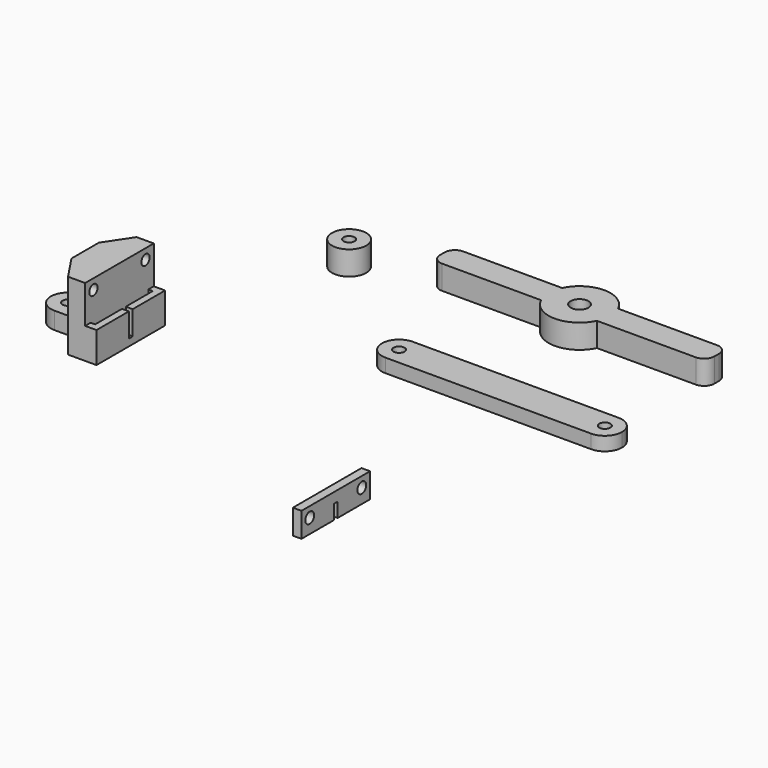
from build123d import *

# Parameters (mm, degrees)
F0_W      = 70
F0_H      = 10
F0_R      = 1.6
F1_DEPTH  = 4
F2_R      = 4.99999
F3_R      = 5
F3_R_2    = 1.6
F4_DEPTH  = 7
F7_DEPTH  = 20
F6_W      = 10
F6_H      = 10
F8_DEPTH  = 5
F10_D     = 3.2
F10_DEPTH = 5
F10_TIP   = 0.9613769904
F11_R     = 4.99999
F13_DEPTH = 1.3
F14_W     = 9.8
F14_H     = 7
F15_DEPTH = 2
F16_D     = 3
F16_DEPTH = 10
F16_TIP   = 0.9012909285
F17_R     = 1.6
F18_DEPTH = 2.5
F5_R      = 2.6
F19_DEPTH = 7
F20_R     = 3


# Not quite as in the source:
# - a fillet or chamfer is up to 0.001 mm smaller than in the source, because OpenCascade refuses the exact size


with BuildPart() as f1:
    # F0 (on Top) → F1 (new body)
    with BuildSketch(Plane.XY):
        with Locations((17.1764425881, -2.1875003539)):
            Rectangle(F0_W, F0_H)
        with Locations((-12.8235574119, -2.1875003539)):
            Circle(F0_R, mode=Mode.SUBTRACT)
        with Locations((47.1764425881, -2.1875003539)):
            Circle(F0_R, mode=Mode.SUBTRACT)
    extrude(amount=F1_DEPTH)

    # F2 (radius 5 in the source; OpenCascade refuses exactly that, so slightly less here)
    f2_edges = [f1.edges().sort_by_distance(p)[0] for p in [
        (-17.823557, 2.8125, 2),
        (-17.823557, -7.1875, 2),
        (52.176443, 2.8125, 2),
        (52.176443, -7.1875, 2),
    ]]
    fillet(f2_edges, radius=F2_R)


with BuildPart() as f4:
    # F3 (on Top) → F4 (new body)
    with BuildSketch(Plane.XY):
        with Locations((-52.1052666008, 28.7171080709)):
            Circle(F3_R)
        with Locations((-52.1052666008, 28.7171080709)):
            Circle(F3_R_2, mode=Mode.SUBTRACT)
    extrude(amount=F4_DEPTH)


with BuildPart() as f7:
    # F6 (on Top) → F7 (new body)
    with BuildSketch(Plane.XY):
        Polygon((-74.9508264661, -20.1742056012), (-79.9508264661, -27.6742056012), (-79.9508264661, -37.6742056012), (-74.9508264661, -45.1742056012), (-69.9508264661, -45.1742056012), (-69.9508264661, -20.1742056012), align=None)
    extrude(amount=F7_DEPTH)

    # F6 (on Top) → F8 (join)
    with BuildSketch(Plane.XY):
        with Locations((-84.9508264661, -32.6742056012)):
            Rectangle(F6_W, F6_H)
    extrude(amount=F8_DEPTH)

    # F10
    with Locations(Plane.XY.offset(5)):
        with Locations((-84.9508264661, -32.6742056012)):
            Hole(F10_D / 2, depth=F10_DEPTH)
            with Locations((0, 0, -(F10_DEPTH + F10_TIP / 2))):  # 118° drill point
                Cone(0, F10_D / 2, F10_TIP, mode=Mode.SUBTRACT)

    # F11 (radius 5 in the source; OpenCascade refuses exactly that, so slightly less here)
    f11_edges = [f7.edges().sort_by_distance(p)[0] for p in [
        (-89.950826, -37.674206, 2.5),
        (-89.950826, -27.674206, 2.5),
    ]]
    fillet(f11_edges, radius=F11_R)

    # F12 (on face) → F13 (join)
    with BuildSketch(Plane.YZ.offset(-69.9508264661)):
        Polygon((-43.1742056012, 9), (-45.1742056012, 9), (-45.1742056012, 0), (-20.1742056012, 0), (-20.1742056012, 9), (-22.1742056012, 9), (-22.1742056012, 2), (-43.1742056012, 2), align=None)
    extrude(amount=F13_DEPTH)

    # F14 (on face) → F15 (join)
    with BuildSketch(Plane.YZ.offset(-68.6508264661)):
        Polygon((-43.1742056012, 9), (-45.1742056012, 9), (-45.1742056012, 0), (-20.1742056012, 0), (-20.1742056012, 9), (-22.1742056012, 9), (-22.1742056012, 2), (-31.9742056012, 2), (-33.3742056012, 2), (-43.1742056012, 2), align=None)
        with Locations((-38.2742056012, 5.5)):
            Rectangle(F14_W, F14_H)
        with Locations((-27.0742056012, 5.5)):
            Rectangle(F14_W, F14_H)
    extrude(amount=F15_DEPTH)

    # F16
    with Locations(Plane.YZ.offset(-69.9508264661)):
        with Locations((-42.1742056012, 17), (-23.1742056012, 17)):
            Hole(F16_D / 2, depth=F16_DEPTH)
            with Locations((0, 0, -(F16_DEPTH + F16_TIP / 2))):  # 118° drill point
                Cone(0, F16_D / 2, F16_TIP, mode=Mode.SUBTRACT)


with BuildPart() as f18:
    # F17 (on Right) → F18 (new body)
    with BuildSketch(Plane.YZ):
        Polygon((-31.9078966975, -10.1387043178), (-56.9078966975, -10.1387043178), (-56.9078966975, -17.3387043178), (-45.1078966975, -17.3387043178), (-45.1078966975, -13.1387043178), (-43.7078966975, -13.1387043178), (-43.7078966975, -17.3387043178), (-31.9078966975, -17.3387043178), align=None)
        with Locations((-53.9078966975, -13.1387043178)):
            Circle(F17_R, mode=Mode.SUBTRACT)
        with Locations((-34.9078966975, -13.1387043178)):
            Circle(F17_R, mode=Mode.SUBTRACT)
    extrude(amount=F18_DEPTH)


with BuildPart() as f19:
    # F5 (on Top) → F19 (new body)
    with BuildSketch(Plane.XY):
        with BuildLine():
            ThreePointArc((0.7788947706, 32.5657874346), (-0.0855284333, 36.4144742489), (0.7788947706, 40.2631610632))
            Line((0.7788947706, 40.2631610632), (-31.0855284333, 40.2631610632))
            Line((-31.0855284333, 40.2631610632), (-31.0855284333, 32.5657874346))
            Line((-31.0855284333, 32.5657874346), (0.7788947706, 32.5657874346))
        make_face()
        with BuildLine():
            ThreePointArc((17.0500483628, 32.5657874346), (17.6957069913, 34.4421901878), (17.9144715667, 36.4144742489))
            ThreePointArc((17.9144715667, 36.4144742489), (17.6957069913, 38.3867583099), (17.0500483628, 40.2631610632))
            Line((17.0500483628, 40.2631610632), (0.7788947706, 40.2631610632))
            ThreePointArc((0.7788947706, 40.2631610632), (-0.0855284333, 36.4144742489), (0.7788947706, 32.5657874346))
            Line((0.7788947706, 32.5657874346), (17.0500483628, 32.5657874346))
        make_face()
        with Locations((8.9144715667, 36.4144742489)):
            Circle(F5_R, mode=Mode.SUBTRACT)
        with BuildLine():
            Line((0.7788947706, 40.2631610632), (17.0500483628, 40.2631610632))
            ThreePointArc((17.0500483628, 40.2631610632), (8.9144715667, 45.4144742489), (0.7788947706, 40.2631610632))
        make_face()
        with BuildLine():
            ThreePointArc((0.7788947706, 32.5657874346), (8.9144715667, 27.4144742489), (17.0500483628, 32.5657874346))
            Line((17.0500483628, 32.5657874346), (0.7788947706, 32.5657874346))
        make_face()
        with BuildLine():
            ThreePointArc((17.0500483628, 40.2631610632), (17.6957069913, 38.3867583099), (17.9144715667, 36.4144742489))
            ThreePointArc((17.9144715667, 36.4144742489), (17.6957069913, 34.4421901878), (17.0500483628, 32.5657874346))
            Line((17.0500483628, 32.5657874346), (48.9144715667, 32.5657874346))
            Line((48.9144715667, 32.5657874346), (48.9144715667, 40.2631610632))
            Line((48.9144715667, 40.2631610632), (17.0500483628, 40.2631610632))
        make_face()
    extrude(amount=F19_DEPTH)

    # F20
    f20_edges = [f19.edges().sort_by_distance(p)[0] for p in [
        (-31.085528, 40.263161, 3.5),
        (-31.085528, 32.565787, 3.5),
        (48.914472, 40.263161, 3.5),
        (48.914472, 32.565787, 3.5),
    ]]
    fillet(f20_edges, radius=F20_R)


solid = Compound([f1.part, f4.part, f7.part, f18.part, f19.part])
